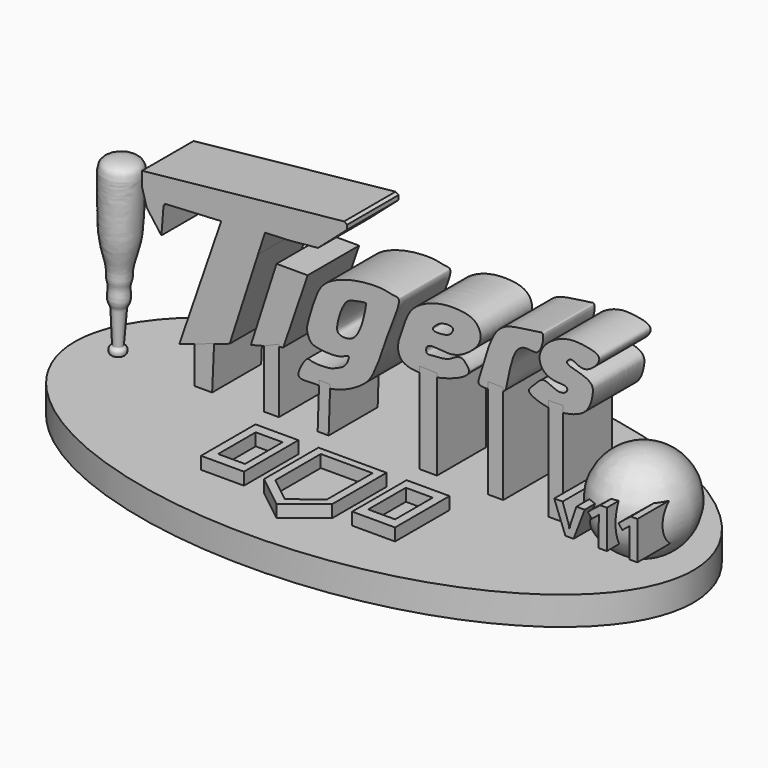
from build123d import *

# Parameters (mm, degrees)
F2_DEPTH      = 4.6
F3_DEPTH      = 10.4
F5_DEPTH      = 9.9
F7_DEPTH      = 2
F6_W          = 6.9349864498
F6_H          = 11
F6_W_2        = 4.3463818729
F6_H_2        = 7.5930785388
F8_DEPTH      = 2
F11_TEXT_SIZE = 8.6544962813
F12_DEPTH     = 9.2


# Not quite as in the source:
# - Text() gives the source's letters only with a copy of the font that has no kerning and outlines rounded to 1/6400 em; it was checked with that copy


with BuildPart() as f2:
    # F0 (on Top) → F2 (new body)
    with BuildSketch(Plane.XY):
        with BuildLine():
            add(Edge.make_bspline(
                [(50, 0), (50, 47.6313972081), (-25, 23.8156986041), (-100, 0), (-25, -23.8156986041), (50, -47.6313972081), (50, 0)],
                knots=[0, 0, 0, 2.0943951024, 2.0943951024, 4.1887902048, 4.1887902048, 6.2831853072, 6.2831853072, 6.2831853072], degree=2, weights=[1, 0.5, 1, 0.5, 1, 0.5, 1]))
        make_face()
    extrude(amount=-F2_DEPTH)

    # F6 (on Top) → F7 (join)
    with BuildSketch(Plane.XY):
        Polygon((5.5, -6.3768545655), (-5.5, -6.3768545655), (-5.5, -17.3768545655), (0, -21.7069815844), (5.5, -17.3768545655), align=None)
        Polygon((-4.1887676343, -16.7122334242), (-4.1887676343, -7.5580496341), (4.1894307213, -7.5580496341), (4.1894307213, -16.7122334242), (0, -20.041026175), align=None, mode=Mode.SUBTRACT)
    extrude(amount=F7_DEPTH)

    # F9 (on Front) → F10 (revolve)
    with BuildSketch(Plane.XZ):
        with BuildLine():
            Line((41.9371388853, 15), (41.9371388853, 0))
            ThreePointArc((41.9371388853, 0), (49.5156368151, 7.5), (41.9371388853, 15))
        make_face()
    revolve(axis=Axis((41.9371388853, 0, 7.5), (0, 0, 1)))

    # F11 (on Front) → F12 (join)
    with BuildSketch(Plane.XZ):
        with Locations((34.8634397153, 4.3135071058)):
            Text('v11', F11_TEXT_SIZE, font='Open Sans', font_style=FontStyle.BOLD, text_align=(TextAlign.LEFT, TextAlign.BOTTOM))
    extrude(amount=F12_DEPTH)


with BuildPart() as f3:
    # F1 (on Front) → F3 (new body)
    with BuildSketch(Plane.XZ):
        Polygon((-38.3655056357, 22.8731110692), (-35.9908305109, 19.6821410209), (-35.6444343925, 24.0251086652), (-35.3967919946, 24.3718065321), (-26.3167731464, 24.8629394919), (-33.0858416855, 5.185410846), (-24.9524656683, 7.8615546227), (-20.3883573413, 22.0222640783), (-19.2411150783, 25.5301780999), (-15.115454793, 25.7066767663), (-10.6588592753, 26.1479243636), (-5.9816408902, 30.2515216172), (-5.9816408902, 30.9575162828), (-6.4492635429, 31.2905423343), (-39.1075909138, 27.8769452125), (-39.1075909138, 27.1772090346), (-39.1075909138, 25.5446210504), align=None)
    extrude(amount=-F3_DEPTH)


with BuildPart() as f3b:
    # F1 (on Front) → F3, piece 2 (new body)
    with BuildSketch(Plane.XZ):
        Polygon((-17.3828210682, 21.6968879104), (-21.5232670307, 8.806255646), (-16.2849724293, 10.1645076647), (-12.3473396525, 21.6968879104), align=None)
    extrude(amount=-F3_DEPTH)


with BuildPart() as f3c:
    # F1 (on Front) → F3, piece 3 (new body)
    with BuildSketch(Plane.XZ):
        with BuildLine():
            add(Edge.make_bspline(
                [(-13.8175217435, 7.021789439), (-13.7054138659, 6.4753410224), (-11.5956343811, 6.7117066042), (-7.9233097006, 6.4833571787), (-3.5212903176, 8.7198824249), (-1.7194282015, 10.7657409981), (-0.0792379792, 15.3673313491), (0.5476525997, 17.5554938855), (3.0700830409, 23.3772626606), (1.5359148423, 23.2855711197), (0.1094304189, 23.8081039865), (-4.1381326086, 23.7683679907), (-8.4005848935, 22.4392579004), (-10.3307199622, 20.8000150028), (-11.1721928173, 18.7400916369), (-11.7752529498, 16.9235735774), (-12.0943249447, 15.739312131), (-12.4918180312, 14.4106044673), (-12.4400843567, 13.5153501375), (-11.9506643723, 12.2255181171), (-10.7999234131, 11.8577445626), (-8.8002739917, 11.6200248051), (-6.85902878, 11.7698703883), (-5.4641614044, 12.6878971454), (-5.9382554711, 11.186534254), (-6.6565479892, 10.4523746546), (-7.8133555039, 9.9485183994), (-8.7921849945, 9.5231435028), (-11.8715960251, 9.494156239), (-12.4113864118, 10.2415407385), (-13.9612797526, 7.7225103716), (-13.8175217435, 7.021789439)],
                knots=[0, 0, 0, 0, 0.032909989, 0.0810167812, 0.1326110556, 0.1727262132, 0.2232934032, 0.2647377294, 0.3199243069, 0.3407665416, 0.3699919709, 0.4191903084, 0.4701707166, 0.5071614626, 0.5424031161, 0.5753153805, 0.6020921578, 0.6296128349, 0.6525114224, 0.6791329575, 0.704416189, 0.7383835475, 0.7732234511, 0.7975352071, 0.8213072304, 0.846833574, 0.8724658031, 0.8986397666, 0.9395009616, 0.9577989111, 1, 1, 1, 1], degree=3))
        make_face()
        with BuildLine():
            add(Edge.make_bspline(
                [(-4.6790586784, 20.555742085), (-5.3305009901, 20.4273011766), (-6.5291171956, 20.2144225532), (-7.9926621592, 15.4418386587), (-6.9814891025, 14.7200913993), (-3.9476035613, 14.5980351733), (-2.8874284969, 20.4657575037), (-2.9145559815, 20.9157160401), (-4.0421696586, 20.6813136096), (-4.6790586784, 20.555742085)],
                knots=[0, 0, 0, 0, 0.1326749483, 0.3410618105, 0.4366976796, 0.5892737405, 0.8202885473, 0.8702890244, 1, 1, 1, 1], degree=3))
        make_face(mode=Mode.SUBTRACT)
    extrude(amount=-F3_DEPTH)


with BuildPart() as f3d:
    # F1 (on Front) → F3, piece 4 (new body)
    with BuildSketch(Plane.XZ):
        with BuildLine():
            add(Edge.make_bspline(
                [(7.0483135059, 17.9219730198), (7.5688616908, 18.3675246707), (10.4843046897, 17.6294400616), (13.2384425996, 18.6873726599), (16.149140054, 21.2739721354), (15.0730850794, 24.2373180198), (12.2926445386, 24.7903530869), (9.9055630713, 24.7882766428), (7.4257354811, 24.2790958599), (4.7753482658, 22.8983463913), (3.5960481135, 20.9461946218), (3.002116658, 19.0341995104), (2.1725300395, 16.9683468615), (2.276601805, 15.0388672303), (3.5445948536, 13.8657472837), (6.3250157048, 13.6347715602), (9.0845113867, 13.9537518822), (12.539198001, 15.0847320409), (14.0018778812, 16.3580731931), (13.3824780006, 17.3098465369), (12.5157212916, 18.335158455), (11.0335966616, 17.5592899297), (10.2792266972, 16.9814131902), (7.6331580936, 16.7856391585), (6.758963515, 16.7408292266), (6.7564549287, 17.6721631565), (7.0483135059, 17.9219730198)],
                knots=[0, 0, 0, 0, 0.0512829803, 0.1028772751, 0.1564496101, 0.201617468, 0.2483367498, 0.2931476589, 0.3390588676, 0.3883244754, 0.431089766, 0.4719581928, 0.5150996607, 0.5536409878, 0.5892169708, 0.636169003, 0.6856733026, 0.741187112, 0.7774384045, 0.8051703116, 0.8364833771, 0.8705576479, 0.9004202437, 0.9470285944, 0.971246893, 1, 1, 1, 1], degree=3))
        make_face()
        with BuildLine():
            add(Edge.make_bspline(
                [(7.9179340973, 20.5738637596), (8.1006778181, 20.2704336638), (10.2343462978, 20.333593967), (10.9902676841, 21.0438160784), (11.3514216447, 22.0619370027), (9.5580016495, 22.0639196206), (8.6165464743, 21.5991282205), (7.7887570623, 20.7883510205), (7.9179340973, 20.5738637596)],
                knots=[0, 0, 0, 0, 0.2175630706, 0.3785149982, 0.5005318124, 0.6754931896, 0.8462100242, 1, 1, 1, 1], degree=3))
        make_face(mode=Mode.SUBTRACT)
    extrude(amount=-F3_DEPTH)


with BuildPart() as f3e:
    # F1 (on Front) → F3, piece 5 (new body)
    with BuildSketch(Plane.XZ):
        with BuildLine():
            add(Edge.make_bspline(
                [(15.4400039464, 15.1570914313), (16.0368250991, 14.8323854039), (19.3728639655, 15.1663324672), (19.8979728343, 16.311623797), (20.7804627406, 22.4632393463), (23.2915933319, 22.9729794276), (25.2859446397, 22.2860227057), (26.0454926284, 26.1212472138), (24.6934197547, 25.6230003137), (20.81786856, 25.3570362195), (17.4122151038, 24.0336951152), (15.6613528772, 16.6599710727), (15.0828967853, 15.3513788608), (15.4400039464, 15.1570914313)],
                knots=[0, 0, 0, 0, 0.102540306, 0.1653150716, 0.2951868223, 0.3742043143, 0.4433858087, 0.534088233, 0.5823120837, 0.6888480171, 0.7912952163, 0.9386451412, 1, 1, 1, 1], degree=3))
        make_face()
    extrude(amount=-F3_DEPTH)


with BuildPart() as f3f:
    # F1 (on Front) → F3, piece 6 (new body)
    with BuildSketch(Plane.XZ):
        with BuildLine():
            add(Edge.make_bspline(
                [(23.4053730965, 16.9133488089), (23.4513920963, 16.5394663439), (25.1536390422, 15.6925953101), (28.2086328227, 15.2358601771), (32.8285714482, 16.2774146459), (33.7364748665, 19.3298914803), (33.9027625195, 21.5818645295), (30.6044693219, 22.3145935496), (29.2110677844, 22.8491851498), (30.4002483112, 24.0340958167), (32.2934274642, 21.913172202), (35.9913695174, 25.4549741771), (32.5443492494, 26.3079450543), (30.0407221717, 26.4746688034), (27.7926134584, 25.7302917313), (25.8638448974, 24.3560841968), (24.7740849374, 22.2052790013), (25.8005760784, 20.0112667439), (27.9723758956, 19.528730046), (29.6257726472, 19.6154487493), (29.6640902584, 18.6378059012), (28.0895017848, 17.9514075834), (25.6793153181, 19.8534245406), (24.4109902201, 17.987538864), (23.3647160762, 17.243667743), (23.4053730965, 16.9133488089)],
                knots=[0, 0, 0, 0, 0.0403206636, 0.0956876367, 0.1582349021, 0.2093225759, 0.2497729062, 0.3030542682, 0.3344622958, 0.3628572938, 0.4074720766, 0.4618608562, 0.5072795556, 0.5571508657, 0.6024501459, 0.6483806302, 0.6930616073, 0.7361915164, 0.7807689831, 0.8166343411, 0.8394755782, 0.8748504237, 0.9228819052, 0.9643773649, 1, 1, 1, 1], degree=3))
        make_face()
    extrude(amount=-F3_DEPTH)


with BuildPart() as f5:
    # F4 (on Front) → F5 (new body)
    with BuildSketch(Plane.XZ):
        Polygon((-27.4745598435, 7.0513123646), (-30.6587219238, 5.9899250045), (-30.6587219238, 0), (-27.7890451252, 0), align=None)
    extrude(amount=-F5_DEPTH)


with BuildPart() as f5b:
    # F4 (on Front) → F5, piece 2 (new body)
    with BuildSketch(Plane.XZ):
        Polygon((-17.0010644943, 10.3932339698), (-19.4128435105, 9.3543129042), (-19.4128435105, 0), (-17.0010644943, 0), align=None)
    extrude(amount=-F5_DEPTH)


with BuildPart() as f5c:
    # F4 (on Front) → F5, piece 3 (new body)
    with BuildSketch(Plane.XZ):
        Polygon((-8.7068295106, 7.3296837509), (-10.4858279228, 7.3852771893), (-10.7359979302, 0), (-8.9570013806, 0), align=None)
    extrude(amount=-F5_DEPTH)


with BuildPart() as f5d:
    # F4 (on Front) → F5, piece 4 (new body)
    with BuildSketch(Plane.XZ):
        Polygon((8.5606537759, 14.5671777427), (5.7375403121, 14.6662341431), (5.7375403121, 0), (8.5606537759, 0), align=None)
    extrude(amount=-F5_DEPTH)


with BuildPart() as f5e:
    # F4 (on Front) → F5, piece 5 (new body)
    with BuildSketch(Plane.XZ):
        Polygon((19.2587673664, 16.0034988075), (16.8318804353, 16.0530265421), (16.8318804353, 0), (19.2587673664, 0), align=None)
    extrude(amount=-F5_DEPTH)


with BuildPart() as f5f:
    # F4 (on Front) → F5, piece 6 (new body)
    with BuildSketch(Plane.XZ):
        Polygon((28.9167873561, 16.5978390723), (26.5889558941, 16.5483094752), (26.5889558941, 0), (28.9167873561, 0), align=None)
    extrude(amount=-F5_DEPTH)


with BuildPart() as f8:
    # F6 (on Top) → F8 (new body)
    with BuildSketch(Plane.XY):
        with Locations((-12.2122108005, -11.8768545655)):
            Rectangle(F6_W, F6_H)
        with Locations((-12.128226459, -11.84888836)):
            Rectangle(F6_W_2, F6_H_2, mode=Mode.SUBTRACT)
    extrude(amount=F8_DEPTH)


with BuildPart() as f8b:
    # F6 (on Top) → F8, piece 2 (new body)
    with BuildSketch(Plane.XY):
        with Locations((12.2122108005, -11.8768545655)):
            Rectangle(F6_W, F6_H)
        with Locations((12.128226459, -11.84888836)):
            Rectangle(F6_W_2, F6_H_2, mode=Mode.SUBTRACT)
    extrude(amount=F8_DEPTH)


with BuildPart() as f14:
    # F13 (on Front) → F14 (revolve)
    with BuildSketch(Plane.XZ):
        with BuildLine():
            Line((-42.3833240844, 28.6985960701), (-43.0364968222, 0.3384350103))
            add(Edge.make_bspline(
                [(-42.3833240844, 28.6985960701), (-42.0629178811, 28.6951766067), (-41.3338518136, 28.6873958125), (-39.2925383304, 28.2327407169), (-39.2958152355, 25.7667557498), (-39.6128145095, 20.9196014281), (-39.8056758295, 16.6401490415), (-41.1466331943, 12.9861949132), (-40.9981113375, 11.3808910192), (-41.5149525122, 10.26582394), (-41.1416400397, 8.57573856), (-41.6657914147, 7.5367415373), (-41.9098109113, 7.1711026313), (-42.0869156001, 2.3220563917), (-42.3403657326, 1.6854108325), (-41.8078474254, 1.5624171604), (-41.7659802611, 0.9648083666), (-41.9275870355, 0.4982153413), (-42.6133739717, 0.3994018355), (-43.0364968222, 0.3384350103)],
                knots=[0, 0, 0, 0, 0.0482411892, 0.1097700786, 0.1772853122, 0.2811628023, 0.3808138344, 0.4712218257, 0.5284639606, 0.578551353, 0.6395429149, 0.6865406504, 0.7204128328, 0.8228792345, 0.8585256289, 0.8871193218, 0.92112304, 0.9513338001, 1, 1, 1, 1], degree=3))
        make_face()
    revolve(axis=Axis((-42.6980312914, 0, 15.0342978537), (0.023025242, 0, 0.999734884)))


solid = Compound([f2.part, f3.part, f3b.part, f3c.part, f3d.part, f3e.part, f3f.part, f5.part, f5b.part, f5c.part, f5d.part, f5e.part, f5f.part, f8.part, f8b.part, f14.part])
